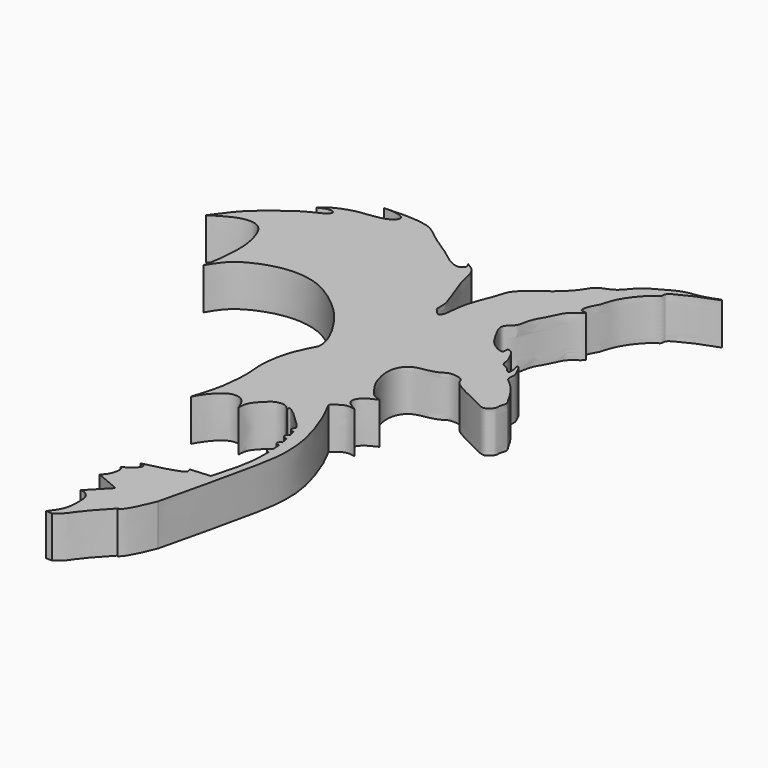
from build123d import *

# Parameters (mm, degrees)
F1_DEPTH = 10


# Not quite as in the source:
# - a feature of the source that left no trace in its solid (it failed there, or was rolled back) is left out


with BuildPart() as f1:
    # F0 (on Top) → F1 (new body)
    with BuildSketch(Plane.XY):
        with BuildLine():
            add(Edge.make_bspline(
                [(-6.6337995231, -72.9357004166), (-7.1314396337, -72.9271546006), (-7.6290797442, -72.9186087847), (-8.1267198548, -72.9100629687)],
                knots=[0, 0, 0, 0, 1.4931404473, 1.4931404473, 1.4931404473, 1.4931404473], degree=3))
            add(Edge.make_bspline(
                [(2.0687442739, -63.2870793343), (1.0655686157, -64.3116531159), (-0.8187090192, -66.313104324), (-4.195089807, -70.2883444329), (-4.627157934, -71.4743211865), (-6.6337995231, -72.9357004166)],
                knots=[0, 0, 0, 0, 0.3335705597, 0.6748681138, 1, 1, 1, 1], degree=3))
            add(Edge.make_bspline(
                [(1.910535153, -63.9636665583), (1.9632715266, -63.7381374836), (2.0160079002, -63.5126084089), (2.0687442739, -63.2870793343)],
                knots=[0, 0, 0, 0, 0.6948383968, 0.6948383968, 0.6948383968, 0.6948383968], degree=3))
            add(Edge.make_bspline(
                [(5.8438498527, -56.6447414458), (5.4905020604, -57.5289442822), (4.7481885513, -59.3864787695), (3.0953195634, -62.6960238518), (2.2510695377, -63.5993167869), (1.910535153, -63.9636665583)],
                knots=[0, 0, 0, 0, 0.3514947842, 0.7384207073, 1, 1, 1, 1], degree=3))
            add(Edge.make_bspline(
                [(6.3076945953, -5.9148361906), (7.0007636236, -7.2003286762), (8.5380538216, -10.0516680335), (10.9089129574, -16.6613939413), (12.0674852767, -21.8304357524), (12.3113407299, -28.8444537858), (9.7604078065, -39.3626024965), (7.7722802305, -49.0731480059), (6.0229022974, -55.3898122234), (5.8847139664, -56.3583361388), (5.8438498527, -56.6447414458)],
                knots=[0, 0, 0, 0, 0.109376109, 0.2426061668, 0.359029114, 0.4906517683, 0.6576995727, 0.8224710199, 0.9475023371, 1, 1, 1, 1], degree=3))
            add(Edge.make_bspline(
                [(11.2524237484, -4.2680497281), (10.4897273671, -4.0987371349), (8.823873074, -3.7289305942), (7.192278365, -5.1463626388), (6.3076945953, -5.9148361906)],
                knots=[0, 0, 0, 0, 0.4578409915, 1, 1, 1, 1], degree=3))
            add(Edge.make_bspline(
                [(12.546222657, 1.679057721), (11.8295178697, 1.3570341716), (10.4462161713, 0.7355011068), (8.848394291, -0.5715527639), (8.3221339067, -2.605622428), (10.1715870047, -3.6548637954), (11.2524237484, -4.2680497281)],
                knots=[0, 0, 0, 0, 0.254730566, 0.4916518362, 0.7029168382, 1, 1, 1, 1], degree=3))
            add(Edge.make_bspline(
                [(20.6570085138, 53.6428168416), (20.4942527628, 53.3830949054), (20.0753023136, 52.7145432802), (17.6149198038, 51.4507716398), (16.4514573676, 48.02232008), (14.6631437802, 45.4643299358), (14.145426845, 43.2748312914), (13.8022135925, 41.2259410146), (11.6603933279, 39.8437249086), (11.9731630683, 37.8695130149), (13.5805005994, 35.0346140154), (14.9416748903, 32.8416392773), (17.5862001087, 31.2482015153), (18.621727352, 31.48145368), (18.4084484269, 32.6321978621), (18.8793709811, 32.765984798), (19.8999213372, 32.3723794016), (20.7276311437, 30.4472264461), (21.3542566107, 29.4088049248), (21.4303884181, 27.5649378316), (22.2879530678, 27.063038919), (23.52702602, 26.5713614051), (23.956498275, 25.5925517266), (24.7405505076, 25.6566108818), (24.4469390451, 27.5678390055), (24.084121719, 28.4707751068), (24.8532708174, 28.4655906967), (25.5187420836, 26.6338098023), (26.316010867, 25.4761996307), (25.72507434, 23.5022784699), (27.0006201729, 22.5865782729), (28.2564908431, 21.4095446807), (29.6812082619, 19.6540035188), (30.8106938727, 18.0536136895), (31.5022239887, 16.4421570953), (32.4179840839, 15.5269532995), (31.6099372723, 13.8149448843), (31.8561528543, 12.9138075227), (31.0359163694, 11.7841275493), (29.781570044, 10.9925579459), (27.5529938798, 12.138917656), (24.4728032039, 13.6885614706), (21.1511660633, 15.2714163253), (19.6125248728, 16.5936502944), (19.532203641, 17.5458217265), (18.4195591736, 18.3682068907), (15.6869045591, 18.4469810547), (14.8455638979, 17.4503210339), (11.9329933916, 16.5653755143), (9.4425018716, 16.3227700404), (7.4385912641, 14.9700284143), (6.3446367392, 12.2468657397), (6.6970870347, 9.1822423829), (7.7149878396, 6.2313605186), (8.8406500462, 4.7193805761), (9.9038869256, 3.1687767279), (10.7838233383, 2.1731320277), (11.9235346774, 1.8536232287), (12.546222657, 1.679057721)],
                knots=[0, 0, 0, 0, 0.0136102916, 0.0352910037, 0.0610325614, 0.0849867567, 0.1050605016, 0.1241879178, 0.1443929012, 0.1621517225, 0.1864685492, 0.2090609333, 0.2321683507, 0.2436805244, 0.256726646, 0.2644754835, 0.2778631127, 0.2971774514, 0.3127508888, 0.3301946743, 0.3431327074, 0.3586611894, 0.371986334, 0.3806894828, 0.3989035661, 0.4111665971, 0.4196162316, 0.4379778345, 0.4544759046, 0.4723652825, 0.4881694729, 0.5061239534, 0.5265069848, 0.5456894914, 0.5634652411, 0.5779431924, 0.595442059, 0.608295768, 0.6235620803, 0.6390288189, 0.6594143958, 0.6852695246, 0.7116264308, 0.7300573455, 0.7422203945, 0.7574426633, 0.779019051, 0.7942411191, 0.8173277508, 0.8391183318, 0.8593410525, 0.8818478433, 0.9057616588, 0.9294935306, 0.9481921685, 0.9664834439, 0.9818273298, 1, 1, 1, 1], degree=3))
            add(Edge.make_bspline(
                [(-8.9372685179, 55.1837384701), (-8.3075877658, 54.8235485187), (-7.0510437685, 54.104780286), (-5.999977441, 52.1290676432), (-5.5331139672, 48.5751617471), (-3.7889016886, 44.7829359386), (-3.1568863535, 42.2593815694), (-2.0705895203, 39.9980545438), (-2.338922341, 37.3055477003), (-1.9806680195, 37.0635265279), (-0.9062354717, 35.7539682414), (-0.3972535917, 35.5695790019), (0.4193054352, 36.7366704388), (0.4329272816, 39.9651389304), (1.5157563478, 44.310149684), (3.5061489993, 48.7853552028), (3.9171563242, 51.3944238754), (7.4560905977, 54.5243485301), (11.3957341461, 57.0449823095), (14.4486169339, 60.6013668852), (15.2922160443, 62.4882932796), (17.1363417228, 63.4628115962), (19.6654953516, 64.2585820671), (21.9561156118, 67.6766007386), (25.6680330024, 69.7476580346), (29.6261368761, 72.0283872386), (33.3116303039, 72.1727199198), (36.2000907849, 73.2242527967), (37.215102537, 73.7168687077), (37.5758618881, 73.4969751909), (36.889795742, 73.2049907083), (33.7227959582, 72.1555195551), (29.9107510403, 70.3689742362), (27.7282504592, 69.1511697224), (27.5235127399, 68.3646677324), (27.5789619125, 67.5501760534), (26.0491168244, 67.0583149711), (22.0245504036, 62.4256886948), (20.9749320046, 58.8649019197), (20.6476406854, 57.5902351927), (19.5876546765, 56.060113998), (18.9546295968, 53.5895564544), (20.1330788688, 53.6264252525), (20.6570085138, 53.6428168416)],
                knots=[0, 0, 0, 0, 0.0228385713, 0.0455749514, 0.0754660742, 0.1077204301, 0.1329466338, 0.1583359266, 0.1827873136, 0.1930696998, 0.2132470824, 0.2234067894, 0.239912938, 0.2679745517, 0.3021140323, 0.3366113277, 0.3616814863, 0.3946758326, 0.429884997, 0.4634178433, 0.4854619541, 0.507189838, 0.5323768338, 0.56355735, 0.5962603264, 0.6295755866, 0.6599708308, 0.6875047264, 0.7033281055, 0.710464107, 0.7209533382, 0.7497880308, 0.7835519573, 0.8073705709, 0.8205196401, 0.8330124869, 0.8511376471, 0.8902740045, 0.9206742992, 0.9379339201, 0.9598518457, 0.9821504338, 1, 1, 1, 1], degree=3))
            add(Edge.make_bspline(
                [(-35.5659276247, 63.1499737501), (-34.116668953, 63.2328988927), (-31.2500549834, 63.3969236984), (-27.0740515254, 63.1440962114), (-23.5345665791, 62.4213475017), (-20.4237068053, 59.4341294863), (-16.4339276228, 57.1826876085), (-13.5523686337, 54.8066431247), (-11.2587466258, 53.3112287788), (-9.3435780497, 53.0733192351), (-8.3704502342, 54.2246030975), (-8.753158598, 54.8721988785), (-8.9372685179, 55.1837384701)],
                knots=[0, 0, 0, 0, 0.1214391918, 0.2402050721, 0.3486181487, 0.4679456407, 0.5934532978, 0.706430374, 0.8022067393, 0.8788737867, 0.9417296837, 1, 1, 1, 1], degree=3))
            add(Edge.make_bspline(
                [(-45.6055998802, 55.3824417293), (-45.060998176, 55.9065033345), (-43.8019299288, 57.1180847922), (-39.7121957856, 58.7773102292), (-36.4823701585, 59.1383716893), (-31.7038468718, 59.7677186387), (-30.0143701847, 62.0324158012), (-32.3252357114, 63.1929116814), (-34.3836520711, 63.1656384501), (-35.5659276247, 63.1499737501)],
                knots=[0, 0, 0, 0, 0.1274900061, 0.2947449802, 0.4474667233, 0.6249333334, 0.7384435404, 0.8497719829, 1, 1, 1, 1], degree=3))
            add(Edge.make_bspline(
                [(-59.890113771, 39.9530529976), (-58.8815564406, 41.4106396758), (-56.879682138, 44.3037873701), (-53.2530888506, 47.8645042929), (-49.1457331561, 50.8693003121), (-46.1046668305, 53.0913597778), (-42.2568282918, 54.5091748871), (-41.7618195813, 56.0629931022), (-43.4100549956, 56.4325175194), (-44.7915842599, 55.7717656287), (-45.6055998802, 55.3824417293)],
                knots=[0, 0, 0, 0, 0.1585433909, 0.314691025, 0.4690007256, 0.6068010487, 0.743674885, 0.8139238817, 0.8903614489, 1, 1, 1, 1], degree=3))
            add(Edge.make_bspline(
                [(-47.5430861115, 23.7839054316), (-47.3148964682, 24.8890934474), (-46.8163605078, 27.303646364), (-46.4198292757, 32.4134070329), (-46.6193064832, 37.0538161617), (-48.8383279381, 43.5756773553), (-54.5703000421, 43.4067739334), (-58.0244191204, 41.164296286), (-59.890113771, 39.9530529976)],
                knots=[0, 0, 0, 0, 0.1399023576, 0.3056508402, 0.4705472861, 0.6518021402, 0.8119257415, 1, 1, 1, 1], degree=3))
            add(Edge.make_bspline(
                [(-10.0335814059, 11.4400079474), (-10.0135861936, 12.0221797283), (-9.9665756188, 13.3909188919), (-11.2413712072, 16.6679243127), (-13.2423953671, 20.0905478984), (-16.2188960867, 24.2034331837), (-21.1177732172, 28.4397042297), (-26.5605485818, 31.8508454546), (-33.66514132, 32.7150511398), (-40.2166512719, 30.817551482), (-45.0076935843, 28.0083659115), (-46.7141849748, 25.165017057), (-47.5430861115, 23.7839054316)],
                knots=[0, 0, 0, 0, 0.0613270654, 0.1441855462, 0.2341443731, 0.3349058095, 0.4490411938, 0.5624300651, 0.6806829767, 0.7976107032, 0.9016926079, 1, 1, 1, 1], degree=3))
            add(Edge.make_bspline(
                [(-15.9717816859, -19.549658522), (-15.7721103543, -18.7416869484), (-15.3345370815, -16.9710433463), (-14.1373313906, -13.3602377823), (-13.7121957506, -9.8469825232), (-13.3538122614, -5.1264872275), (-14.083910886, -0.726659679), (-12.9631334683, 5.3845368229), (-11.3684930395, 9.0238933488), (-10.4472297679, 10.6913277944), (-10.0335814059, 11.4400079474)],
                knots=[0, 0, 0, 0, 0.1023711365, 0.2243430386, 0.3444294576, 0.4796541622, 0.614593261, 0.7709340605, 0.8971491065, 1, 1, 1, 1], degree=3))
            add(Edge.make_bspline(
                [(-6.2214001082, -17.3607971519), (-6.4879714832, -16.648761399), (-7.0079314493, -15.2599022765), (-8.598840077, -13.7183492341), (-11.5793677871, -13.7075580627), (-14.6515199377, -17.1283619643), (-15.5670026778, -18.8073132861), (-15.9717816859, -19.549658522)],
                knots=[0, 0, 0, 0, 0.1800787823, 0.3512521085, 0.5459073729, 0.7992237809, 1, 1, 1, 1], degree=3))
            add(Edge.make_bspline(
                [(1.6916047316, -12.7206239849), (1.3963637237, -12.327045556), (0.822465665, -11.5619963579), (-0.351931414, -10.8930673675), (-2.5199442317, -11.1616568485), (-4.0541138902, -12.7016107951), (-6.1742605231, -14.9650596583), (-6.2063799262, -16.5974384358), (-6.2214001082, -17.3607971519)],
                knots=[0, 0, 0, 0, 0.1413764937, 0.2748117407, 0.4410484011, 0.6165731985, 0.8206959102, 1, 1, 1, 1], degree=3))
            add(Edge.make_bspline(
                [(7.4255969375, -17.0555468649), (7.1327909266, -16.6175073864), (6.5311527172, -15.700372042), (4.2437209099, -13.8392435483), (3.4013939405, -12.6554736022), (0.7757052663, -11.0121192411), (1.6916047316, -12.7206239849)],
                knots=[0, 0, 0, 0, 0.2299664628, 0.5224336057, 0.8232235654, 1, 1, 1, 1], degree=3))
            add(Edge.make_bspline(
                [(7.9716136679, -18.5350757092), (7.1437819861, -18.7288243324), (6.5801516175, -17.971444875), (7.4255969375, -17.0555468649)],
                knots=[0, 0, 0, 0, 1.5770668569, 1.5770668569, 1.5770668569, 1.5770668569], degree=3))
            add(Edge.make_bspline(
                [(8.3840126172, -20.0362410396), (8.2465463007, -19.5358525962), (8.1090799843, -19.0354641527), (7.9716136679, -18.5350757092)],
                knots=[0, 0, 0, 0, 1.5567820151, 1.5567820151, 1.5567820151, 1.5567820151], degree=3))
            add(Edge.make_bspline(
                [(8.7803145871, -21.639065817), (7.8203827143, -21.8240059912), (7.2303316556, -20.5910652876), (8.3840126172, -20.0362410396)],
                knots=[0, 0, 0, 0, 1.6510913113, 1.6510913113, 1.6510913113, 1.6510913113], degree=3))
            add(Edge.make_bspline(
                [(9.0885506943, -23.2683084905), (8.9858053252, -22.7252275993), (8.8830599561, -22.1821467082), (8.7803145871, -21.639065817)],
                knots=[0, 0, 0, 0, 1.6581438982, 1.6581438982, 1.6581438982, 1.6581438982], degree=3))
            add(Edge.make_bspline(
                [(9.2999115586, -24.6157385409), (8.2078780979, -24.6773846447), (8.155037649, -23.5765445977), (9.0885506943, -23.2683084905)],
                knots=[0, 0, 0, 0, 1.3639065788, 1.3639065788, 1.3639065788, 1.3639065788], degree=3))
            add(Edge.make_bspline(
                [(9.4496263191, -26.500377804), (9.3997213989, -25.8721647163), (9.3498164788, -25.2439516286), (9.2999115586, -24.6157385409)],
                knots=[0, 0, 0, 0, 1.8905765421, 1.8905765421, 1.8905765421, 1.8905765421], degree=3))
            add(Edge.make_bspline(
                [(9.5307920128, -27.9701855034), (8.4192389622, -27.8301928192), (8.4192389622, -26.8966797739), (9.4496263191, -26.500377804)],
                knots=[0, 0, 0, 0, 1.4720470586, 1.4720470586, 1.4720470586, 1.4720470586], degree=3))
            add(Edge.make_bspline(
                [(7.1534165181, -42.3810631037), (7.5387822477, -41.0268112357), (8.3543865107, -38.1606155361), (9.5481299231, -32.8110731381), (9.5364556586, -29.5515221314), (9.5307920128, -27.9701855034)],
                knots=[0, 0, 0, 0, 0.3156131543, 0.6679769746, 1, 1, 1, 1], degree=3))
            add(Edge.make_bspline(
                [(2.3777191527, -42.7790395916), (3.9696182745, -42.6463807623), (5.5615173963, -42.513721933), (7.1534165181, -42.3810631037)],
                knots=[0, 0, 0, 0, 4.7922511006, 4.7922511006, 4.7922511006, 4.7922511006], degree=3))
            add(Edge.make_bspline(
                [(-6.4270100556, -46.6113202274), (-5.719845311, -46.4233782223), (-4.2147855956, -46.02338099), (-1.4508825274, -45.474812067), (1.2450024562, -44.5800355869), (2.784958523, -43.8733620053), (2.5051825482, -43.1215557155), (2.3777191527, -42.7790395916)],
                knots=[0, 0, 0, 0, 0.2123071486, 0.4518536013, 0.6952683913, 0.8611670441, 1, 1, 1, 1], degree=3))
            add(Edge.make_bspline(
                [(-8.5007091984, -50.09675771), (-8.0215904662, -49.8802250683), (-7.0869114226, -49.4578067641), (-6.03469723, -48.5572094741), (-5.2830769508, -47.5924067528), (-5.3237984117, -46.7178442412), (-6.032694853, -46.6493945519), (-6.4270100556, -46.6113202274)],
                knots=[0, 0, 0, 0, 0.2338424645, 0.4561868204, 0.6613520373, 0.811631104, 1, 1, 1, 1], degree=3))
            add(Edge.make_bspline(
                [(-9.5872869715, -54.9654923379), (-9.1974080523, -54.605478743), (-8.3724491434, -53.8437129539), (-7.7558824666, -51.8926362263), (-7.750164582, -50.5907718583), (-8.2669857593, -50.250596247), (-8.5007091984, -50.09675771)],
                knots=[0, 0, 0, 0, 0.2723420793, 0.5762584575, 0.8083702159, 1, 1, 1, 1], degree=3))
            add(Edge.make_bspline(
                [(-3.7709935568, -57.4315041304), (-4.7727041112, -56.980058634), (-6.7422768548, -56.0924222394), (-8.6498780474, -55.336807062), (-9.5872869715, -54.9654923379)],
                knots=[0, 0, 0, 0, 0.5085928193, 1, 1, 1, 1], degree=3))
            add(Edge.make_bspline(
                [(-8.3884447813, -62.2081123292), (-7.5697734385, -61.3608011599), (-5.9729634226, -59.7081294575), (-4.4924566846, -58.1774277031), (-3.7709935568, -57.4315041304)],
                knots=[0, 0, 0, 0, 0.5126917634, 1, 1, 1, 1], degree=3))
            add(Edge.make_bspline(
                [(-8.1267198548, -72.9100629687), (-7.5535525531, -72.1387716156), (-6.4377957793, -70.6344579002), (-5.6560799225, -68.178261896), (-5.7599838843, -65.5878403158), (-5.7803858078, -63.3309993309), (-7.4045318179, -62.1458403766), (-8.3884447813, -62.2081123292)],
                knots=[0, 0, 0, 0, 0.2117211896, 0.4118607254, 0.6138568456, 0.7981350183, 1, 1, 1, 1], degree=3))
        make_face()
    extrude(amount=F1_DEPTH)


solid = f1.part
